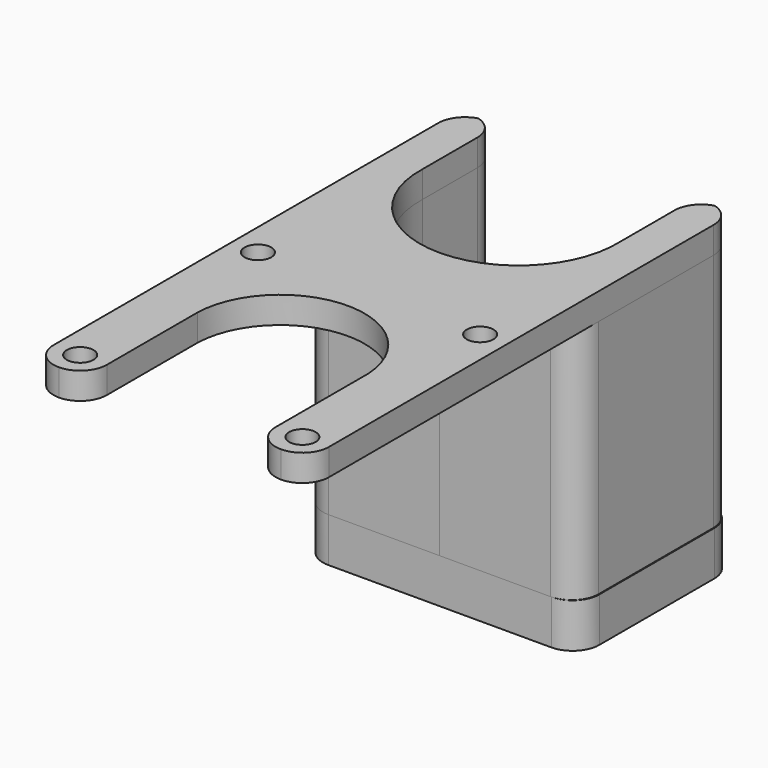
from build123d import *

# Parameters (mm, degrees)
F0_R          = 1.5
F1_DEPTH      = 3
F3_DEPTH      = 27
F5_DEPTH      = 5
F6_F1_R       = 3
F6_F2_R       = 3
F6_2_T1_DEPTH = 42
F6_3_T1_DEPTH = 18
F6_4_T1_DEPTH = 42


# Not quite as in the source:
# - a fillet or chamfer that OpenCascade refuses, or shapes differently, is made with other operations: its cross-section is extruded or revolved along the edge and cut away or added


with BuildPart() as f1:
    # F0 (on Top) → F1 (new body)
    with BuildSketch(Plane.XY):
        with BuildLine():
            Line((-11.0926671237, 57.1), (-15.5, 57.1))
            Line((-15.5, 57.1), (-15.5, 0))
            ThreePointArc((-15.5, 0), (-14.6213203436, -2.1213203436), (-12.5, -3))
            Line((-12.5, -3), (-12.4973975552, -3))
            ThreePointArc((-12.4973975552, -3), (-10.3760772117, -2.1213203436), (-9.4973975552, 0))
            Line((-9.4973975552, 0), (-9.4973975552, 12.2776496511))
            ThreePointArc((-9.4973975552, 12.2776496511), (-9.5, 12.5), (-9.4973975552, 12.7223503489))
            ThreePointArc((-9.4973975552, 12.7223503489), (-0.1600853698, 21.9986510976), (9.4845111786, 13.0422616551))
            ThreePointArc((9.4845111786, 13.0422616551), (9.5, 12.5), (9.4845111786, 11.9577383449))
            Line((9.4845111786, 11.9577383449), (9.4845111786, 0))
            ThreePointArc((9.4845111786, 0), (10.3631908351, -2.1213203436), (12.4845111786, -3))
            Line((12.4845111786, -3), (12.5, -3))
            ThreePointArc((12.5, -3), (14.6213203436, -2.1213203436), (15.5, 0))
            Line((15.5, 0), (15.5, 57.1))
            Line((15.5, 57.1), (11.0886831726, 57.1))
            Line((11.0886831726, 57.1), (11.0886831726, 46.5011042794))
            ThreePointArc((11.0886831726, 46.5011042794), (0.0488899344, 34.9001076683), (-11.0926671237, 46.4034056054))
            Line((-11.0926671237, 46.4034056054), (-11.0926671237, 57.1))
        make_face()
        with Locations((-12.5, 0)):
            Circle(F0_R, mode=Mode.SUBTRACT)
        with Locations((-12.5, 25)):
            Circle(F0_R, mode=Mode.SUBTRACT)
        with Locations((12.5, 0)):
            Circle(F0_R, mode=Mode.SUBTRACT)
        with Locations((12.5, 25)):
            Circle(F0_R, mode=Mode.SUBTRACT)
        with BuildLine():
            ThreePointArc((-9.4973975552, 12.7223503489), (-9.5, 12.5), (-9.4973975552, 12.2776496511))
            Line((-9.4973975552, 12.2776496511), (-9.4973975552, 12.7223503489))
        make_face()
        with BuildLine():
            ThreePointArc((9.4845111786, 11.9577383449), (9.5, 12.5), (9.4845111786, 13.0422616551))
            Line((9.4845111786, 13.0422616551), (9.4845111786, 11.9577383449))
        make_face()
    extrude(amount=F1_DEPTH)

    # F6#3: fillet of radius 3 on 4 edges, made by hand

    # F6_3_s2 → F6_3_t1 (cut)
    with BuildSketch(Plane.XY.offset(-7.5)):
        with BuildLine():
            ThreePointArc((-12.5, 57.1), (-14.6213203436, 56.2213203436), (-15.5, 54.1))
            Line((-15.5, 54.1), (-15.5, 57.1))
            Line((-15.5, 57.1), (-12.5, 57.1))
        make_face()
        with BuildLine():
            ThreePointArc((-11.0926671237, 54.1), (-11.9713467802, 56.2213203436), (-14.0926671237, 57.1))
            Line((-14.0926671237, 57.1), (-11.0926671237, 57.1))
            Line((-11.0926671237, 57.1), (-11.0926671237, 54.1))
        make_face()
        with BuildLine():
            ThreePointArc((14.0886831726, 57.1), (11.967362829, 56.2213203436), (11.0886831726, 54.1))
            Line((11.0886831726, 54.1), (11.0886831726, 57.1))
            Line((11.0886831726, 57.1), (14.0886831726, 57.1))
        make_face()
        with BuildLine():
            ThreePointArc((15.5, 54.1), (14.6213203436, 56.2213203436), (12.5, 57.1))
            Line((12.5, 57.1), (15.5, 57.1))
            Line((15.5, 57.1), (15.5, 54.1))
        make_face()
    extrude(amount=F6_3_T1_DEPTH, mode=Mode.SUBTRACT)


with BuildPart() as f3:
    # F2 (on face) → F3 (new body)
    with BuildSketch(Plane(origin=(0, 0, 0), x_dir=(1, 0, 0), z_dir=(0, 0, -1))):
        with BuildLine():
            ThreePointArc((-11.0926671237, -46.4034056054), (-7.9902378632, -38.2950600982), (0, -34.9))
            Line((0, -34.9), (-12.5, -34.9))
            ThreePointArc((-12.5, -34.9), (-14.6213203436, -35.7786796564), (-15.5, -37.9))
            Line((-15.5, -37.9), (-15.5, -57.1))
            Line((-15.5, -57.1), (-11.0926671237, -57.1))
            Line((-11.0926671237, -57.1), (-11.0926671237, -46.4034056054))
        make_face()
    extrude(amount=F3_DEPTH)

    # F6#2: fillet of radius 3 on 2 edges, made by hand

    # F6_2_s2 → F6_2_t1 (cut)
    with BuildSketch(Plane.XY.offset(-34.5)):
        with BuildLine():
            ThreePointArc((-15.5, 54.1), (-14.6213203436, 56.2213203436), (-12.5, 57.1))
            Line((-12.5, 57.1), (-15.5, 57.1))
            Line((-15.5, 57.1), (-15.5, 54.1))
        make_face()
        with BuildLine():
            ThreePointArc((-14.0926671237, 57.1), (-11.9713467802, 56.2213203436), (-11.0926671237, 54.1))
            Line((-11.0926671237, 54.1), (-11.0926671237, 57.1))
            Line((-11.0926671237, 57.1), (-14.0926671237, 57.1))
        make_face()
    extrude(amount=F6_2_T1_DEPTH, mode=Mode.SUBTRACT)


with BuildPart() as f3b:
    # F2 (on face) → F3, piece 2 (new body)
    with BuildSketch(Plane(origin=(0, 0, 0), x_dir=(1, 0, 0), z_dir=(0, 0, -1))):
        with BuildLine():
            Line((12.5, -34.9), (0, -34.9))
            ThreePointArc((0, -34.9), (8.0240967561, -38.3303278265), (11.0886831726, -46.5011042794))
            Line((11.0886831726, -46.5011042794), (11.0886831726, -57.1))
            Line((11.0886831726, -57.1), (15.5, -57.1))
            Line((15.5, -57.1), (15.5, -37.9))
            ThreePointArc((15.5, -37.9), (14.6213203436, -35.7786796564), (12.5, -34.9))
        make_face()
    extrude(amount=F3_DEPTH)

    # F6#4: fillet of radius 3 on 2 edges, made by hand

    # F6_4_s2 → F6_4_t1 (cut)
    with BuildSketch(Plane.XY.offset(-34.5)):
        with BuildLine():
            ThreePointArc((11.0886831726, 54.1), (11.967362829, 56.2213203436), (14.0886831726, 57.1))
            Line((14.0886831726, 57.1), (11.0886831726, 57.1))
            Line((11.0886831726, 57.1), (11.0886831726, 54.1))
        make_face()
        with BuildLine():
            ThreePointArc((12.5, 57.1), (14.6213203436, 56.2213203436), (15.5, 54.1))
            Line((15.5, 54.1), (15.5, 57.1))
            Line((15.5, 57.1), (12.5, 57.1))
        make_face()
    extrude(amount=F6_4_T1_DEPTH, mode=Mode.SUBTRACT)


with BuildPart() as f5:
    # F4 (on face) → F5 (new body)
    with BuildSketch(Plane(origin=(0, 0, -27), x_dir=(1, 0, 0), z_dir=(0, 0, -1))):
        with BuildLine():
            ThreePointArc((-5.9933118892, -46.2832182873), (0.0601922838, -40.0003019335), (5.9864232992, -46.4034056054))
            Line((5.9864232992, -46.4034056054), (5.9864232992, -54.1))
            ThreePointArc((5.9864232992, -54.1), (6.8651029557, -56.2213203436), (8.9864232992, -57.1))
            Line((8.9864232992, -57.1), (15.5851934105, -57.1))
            Line((15.5851934105, -57.1), (15.5851934105, -37.9))
            ThreePointArc((15.5851934105, -37.9), (14.7065137541, -35.7786796564), (12.5851934105, -34.9))
            Line((12.5851934105, -34.9), (0, -34.9))
            Line((0, -34.9), (-12.5, -34.9))
            ThreePointArc((-12.5, -34.9), (-14.6213203436, -35.7786796564), (-15.5, -37.9))
            Line((-15.5, -37.9), (-15.5, -57.1))
            Line((-15.5, -57.1), (-8.9933118892, -57.1))
            ThreePointArc((-8.9933118892, -57.1), (-6.8719915457, -56.2213203436), (-5.9933118892, -54.1))
            Line((-5.9933118892, -54.1), (-5.9933118892, -46.2832182873))
        make_face()
    extrude(amount=F5_DEPTH)

    # F6: fillet of radius 3 on 2 edges, made by hand

    # F6_f1
    f6_f1_edges = [f5.edges().sort_by_distance(p)[0] for p in [
        (15.5851934105, 57.1, -29.5),
    ]]
    fillet(f6_f1_edges, radius=F6_F1_R)

    # F6_f2
    f6_f2_edges = [f5.edges().sort_by_distance(p)[0] for p in [
        (-15.5, 57.1, -29.5),
    ]]
    fillet(f6_f2_edges, radius=F6_F2_R)


solid = Compound([f1.part, f3.part, f3b.part, f5.part])
